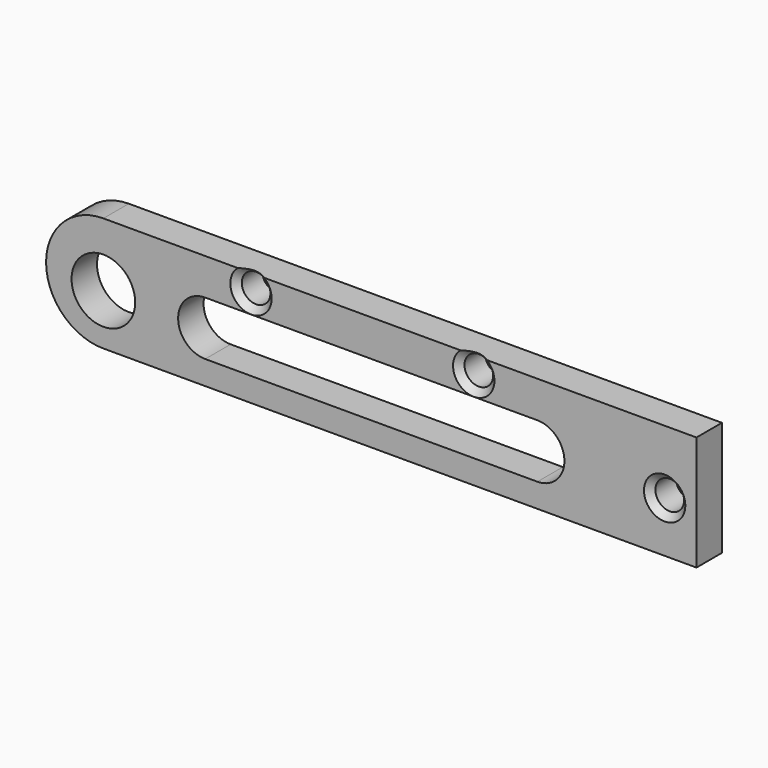
from build123d import *

# Parameters (mm, degrees)
F0_R     = 5
F0_R_2   = 2.25
F1_DEPTH = 5


# Not quite as in the source:
# - a fillet or chamfer that OpenCascade refuses, or shapes differently, is made with other operations: its cross-section is extruded or revolved along the edge and cut away or added


with BuildPart() as f1:
    # F0 (on Front) → F1 (new body)
    with BuildSketch(Plane.XZ):
        with BuildLine():
            Line((54.5685509182, 10), (-38.6314490818, 10))
            ThreePointArc((-38.6314490818, 10), (-47.6314490818, 1), (-38.6314490818, -8))
            Line((-38.6314490818, -8), (54.5685509182, -8))
            Line((54.5685509182, -8), (54.5685509182, 10))
        make_face()
        with Locations((-38.6314490818, 0)):
            Circle(F0_R, mode=Mode.SUBTRACT)
        with BuildLine():
            ThreePointArc((-22.6314490818, -4.25), (-26.8814490818, 0), (-22.6314490818, 4.25))
            Line((-22.6314490818, 4.25), (29.5685509182, 4.25))
            ThreePointArc((29.5685509182, 4.25), (33.8185509182, 0), (29.5685509182, -4.25))
            Line((29.5685509182, -4.25), (-22.6314490818, -4.25))
        make_face(mode=Mode.SUBTRACT)
        with Locations((49.5685509182, 0)):
            Circle(F0_R_2, mode=Mode.SUBTRACT)
        with Locations((-15.4314490818, 7.5)):
            Circle(F0_R_2, mode=Mode.SUBTRACT)
        with Locations((19.5685509182, 7.5)):
            Circle(F0_R_2, mode=Mode.SUBTRACT)
    extrude(amount=F1_DEPTH)

    # F2: chamfer of 1 on 3 edges, made by hand

    # F2_s1 → F2_t2 (revolve, cut)
    with BuildSketch(Plane.XY.offset(7.5)):
        Polygon((-13.1814490818, -4), (-12.1814490818, -5), (-13.1814490818, -5), align=None)
    revolve(axis=Axis((-15.4314490818, -5, 7.5), (0, -1, 0)), mode=Mode.SUBTRACT)

    # F2_s3 → F2_t4 (revolve, cut)
    with BuildSketch(Plane.XY.offset(7.5)):
        Polygon((21.8185509182, -4), (22.8185509182, -5), (21.8185509182, -5), align=None)
    revolve(axis=Axis((19.5685509182, -5, 7.5), (0, -1, 0)), mode=Mode.SUBTRACT)

    # F2_s5 → F2_t6 (revolve, cut)
    with BuildSketch(Plane.XY):
        Polygon((51.8185509182, -4), (52.8185509182, -5), (51.8185509182, -5), align=None)
    revolve(axis=Axis((49.5685509182, -5, 0), (0, -1, 0)), mode=Mode.SUBTRACT)


solid = f1.part
